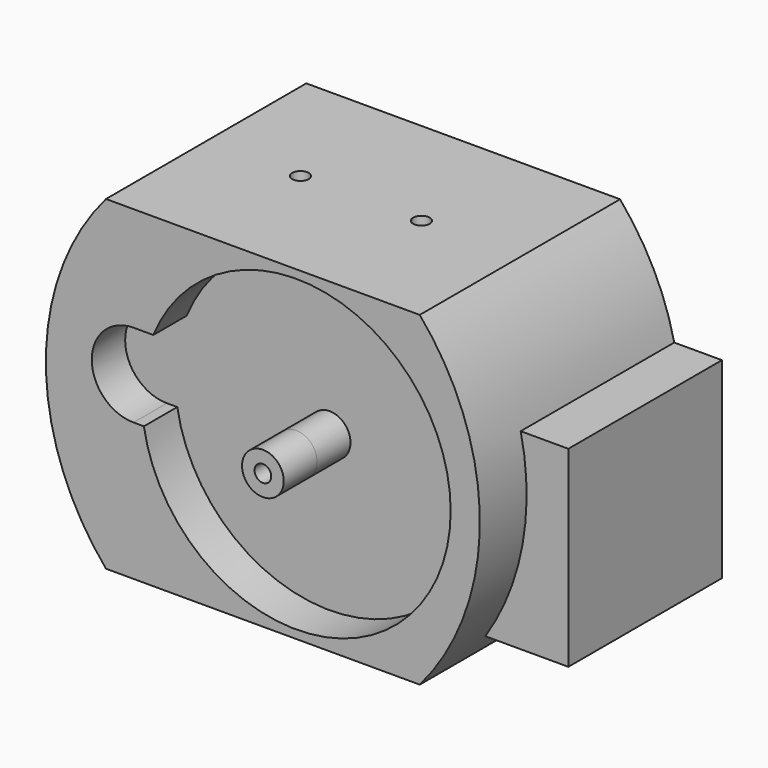
from build123d import *

# Parameters (mm, degrees)
F0_R      = 2.5
F1_DEPTH  = 30
F2_DEPTH  = 5
F3_DEPTH  = 5
F4_R      = 1
F5_DEPTH  = 5
F7_DEPTH  = 23
F8_DEPTH  = 4
F9_R      = 1
F10_DEPTH = 5
F11_R     = 1
F12_DEPTH = 5


# Not quite as in the source:
# - a pattern or mirror of a feature is missing from the dataset's text; its kind, count and spacing are read off the source's solid


with BuildPart() as f1:
    # F0 (on Front) → F1 (new body)
    with BuildSketch(Plane.XZ):
        with BuildLine():
            Line((14.7980262304, 19.5), (-22.7980262304, 19.5))
            ThreePointArc((-22.7980262304, 19.5), (-30, 0), (-22.7980262304, -19.5))
            Line((-22.7980262304, -19.5), (14.7980262304, -19.5))
            ThreePointArc((14.7980262304, -19.5), (22, 0), (14.7980262304, 19.5))
        make_face()
        with BuildLine():
            ThreePointArc((-17.1245437895, 7), (3.5669272416, 18.1528793874), (18.5, 0))
            ThreePointArc((18.5, 0), (1.5049882267, -18.4386824485), (-18.2551362635, -3))
            Line((-18.2551362635, -3), (-19.5, -3))
            ThreePointArc((-19.5, -3), (-24.5, 2), (-19.5, 7))
            Line((-19.5, 7), (-17.1245437895, 7))
        make_face(mode=Mode.SUBTRACT)
        with BuildLine():
            ThreePointArc((-18.2551362635, -3), (1.5049882267, -18.4386824485), (18.5, 0))
            ThreePointArc((18.5, 0), (3.5669272416, 18.1528793874), (-17.1245437895, 7))
            ThreePointArc((-17.1245437895, 7), (-17.2243437117, 6.7507024597), (-17.320514605, 6.4999826014))
            ThreePointArc((-17.320514605, 6.4999826014), (-15.2634077978, 4.6554258627), (-14.5, 2))
            ThreePointArc((-14.5, 2), (-15.5564468025, -1.0738230558), (-18.2793552714, -2.8487138961))
            ThreePointArc((-18.2793552714, -2.8487138961), (-18.2674023824, -2.9243820202), (-18.2551362635, -3))
        make_face()
        Circle(F0_R, mode=Mode.SUBTRACT)
        with BuildLine():
            ThreePointArc((-18.2793552714, -2.8487138961), (-18.4034566143, 1.8875340117), (-17.320514605, 6.4999826014))
            ThreePointArc((-17.320514605, 6.4999826014), (-18.3819465592, 6.8733927098), (-19.5, 7))
            ThreePointArc((-19.5, 7), (-24.5, 2), (-19.5, -3))
            ThreePointArc((-19.5, -3), (-18.885007919, -2.9620343349), (-18.2793552714, -2.8487138961))
        make_face()
        with BuildLine():
            ThreePointArc((-14.5, 2), (-15.2634077978, 4.6554258627), (-17.320514605, 6.4999826014))
            ThreePointArc((-17.320514605, 6.4999826014), (-18.4034566143, 1.8875340117), (-18.2793552714, -2.8487138961))
            ThreePointArc((-18.2793552714, -2.8487138961), (-15.5564468025, -1.0738230558), (-14.5, 2))
        make_face()
        with BuildLine():
            ThreePointArc((-17.320514605, 6.4999826014), (-17.2243437117, 6.7507024597), (-17.1245437895, 7))
            Line((-17.1245437895, 7), (-19.5, 7))
            ThreePointArc((-19.5, 7), (-18.3819465592, 6.8733927098), (-17.320514605, 6.4999826014))
        make_face()
        with BuildLine():
            Line((-19.5, -3), (-18.2551362635, -3))
            ThreePointArc((-18.2551362635, -3), (-18.2674023824, -2.9243820202), (-18.2793552714, -2.8487138961))
            ThreePointArc((-18.2793552714, -2.8487138961), (-18.885007919, -2.9620343349), (-19.5, -3))
        make_face()
        Circle(F0_R)
    extrude(amount=-F1_DEPTH)

    # F0 (on Front) → F2 (cut)
    with BuildSketch(Plane.XZ):
        with BuildLine():
            ThreePointArc((-18.2551362635, -3), (1.5049882267, -18.4386824485), (18.5, 0))
            ThreePointArc((18.5, 0), (3.5669272416, 18.1528793874), (-17.1245437895, 7))
            ThreePointArc((-17.1245437895, 7), (-17.2243437117, 6.7507024597), (-17.320514605, 6.4999826014))
            ThreePointArc((-17.320514605, 6.4999826014), (-15.2634077978, 4.6554258627), (-14.5, 2))
            ThreePointArc((-14.5, 2), (-15.5564468025, -1.0738230558), (-18.2793552714, -2.8487138961))
            ThreePointArc((-18.2793552714, -2.8487138961), (-18.2674023824, -2.9243820202), (-18.2551362635, -3))
        make_face()
        Circle(F0_R, mode=Mode.SUBTRACT)
        with BuildLine():
            ThreePointArc((-17.320514605, 6.4999826014), (-17.2243437117, 6.7507024597), (-17.1245437895, 7))
            Line((-17.1245437895, 7), (-19.5, 7))
            ThreePointArc((-19.5, 7), (-18.3819465592, 6.8733927098), (-17.320514605, 6.4999826014))
        make_face()
        with BuildLine():
            Line((-19.5, -3), (-18.2551362635, -3))
            ThreePointArc((-18.2551362635, -3), (-18.2674023824, -2.9243820202), (-18.2793552714, -2.8487138961))
            ThreePointArc((-18.2793552714, -2.8487138961), (-18.885007919, -2.9620343349), (-19.5, -3))
        make_face()
        with BuildLine():
            ThreePointArc((-18.2793552714, -2.8487138961), (-18.4034566143, 1.8875340117), (-17.320514605, 6.4999826014))
            ThreePointArc((-17.320514605, 6.4999826014), (-18.3819465592, 6.8733927098), (-19.5, 7))
            ThreePointArc((-19.5, 7), (-24.5, 2), (-19.5, -3))
            ThreePointArc((-19.5, -3), (-18.885007919, -2.9620343349), (-18.2793552714, -2.8487138961))
        make_face()
        with BuildLine():
            ThreePointArc((-14.5, 2), (-15.2634077978, 4.6554258627), (-17.320514605, 6.4999826014))
            ThreePointArc((-17.320514605, 6.4999826014), (-18.4034566143, 1.8875340117), (-18.2793552714, -2.8487138961))
            ThreePointArc((-18.2793552714, -2.8487138961), (-15.5564468025, -1.0738230558), (-14.5, 2))
        make_face()
    extrude(amount=-F2_DEPTH, mode=Mode.SUBTRACT)

    # F0 (on Front) → F3 (join)
    with BuildSketch(Plane.XZ):
        Circle(F0_R)
    extrude(amount=F3_DEPTH)

    # F4 (on face) → F5 (cut)
    with BuildSketch(Plane.XY.offset(19.5)):
        with Locations((-11.5, 15)):
            Circle(F4_R)
        with Locations((3, 15)):
            Circle(F4_R)
    f5 = extrude(amount=-F5_DEPTH, mode=Mode.SUBTRACT)

    # F5_copies: F5 across plane
    add(f5.mirror(Plane(origin=(0, 0, 0), x_dir=(-1, 0, 0), z_dir=(0, 0, -1))), mode=Mode.SUBTRACT)

    # F6 (on face) → F7 (join)
    with BuildSketch(Plane(origin=(0, 30, 0), x_dir=(-1, 0, 0), z_dir=(0, 1, 0))):
        with BuildLine():
            Line((-27, -16.5), (-17.0549396327, -16.5))
            ThreePointArc((-17.0549396327, -16.5), (-21.5046036204, -5.4293982359), (-21.2873692912, 6.5))
            Line((-21.2873692912, 6.5), (-27, 6.5))
            Line((-27, 6.5), (-27, -16.5))
        make_face()
    extrude(amount=-F7_DEPTH)

    # F6 (on face) → F8 (join)
    with BuildSketch(Plane(origin=(0, 30, 0), x_dir=(-1, 0, 0), z_dir=(0, 1, 0))):
        with BuildLine():
            ThreePointArc((0, 2.5), (-2.5, 0), (0, -2.5))
            Line((0, -2.5), (0, 2.5))
        make_face()
        with BuildLine():
            Line((0, 2.5), (0, -2.5))
            ThreePointArc((0, -2.5), (1.767766953, -1.767766953), (2.5, 0))
            ThreePointArc((2.5, 0), (1.767766953, 1.767766953), (0, 2.5))
        make_face()
    extrude(amount=F8_DEPTH)

    # F9 (on face) → F10 (cut)
    with BuildSketch(Plane.XZ.offset(5)):
        Circle(F9_R)
    extrude(amount=-F10_DEPTH, mode=Mode.SUBTRACT)

    # F11 (on face) → F12 (cut)
    with BuildSketch(Plane(origin=(0, 34, 0), x_dir=(-1, 0, 0), z_dir=(0, 1, 0))):
        Circle(F11_R)
    extrude(amount=-F12_DEPTH, mode=Mode.SUBTRACT)


solid = f1.part
